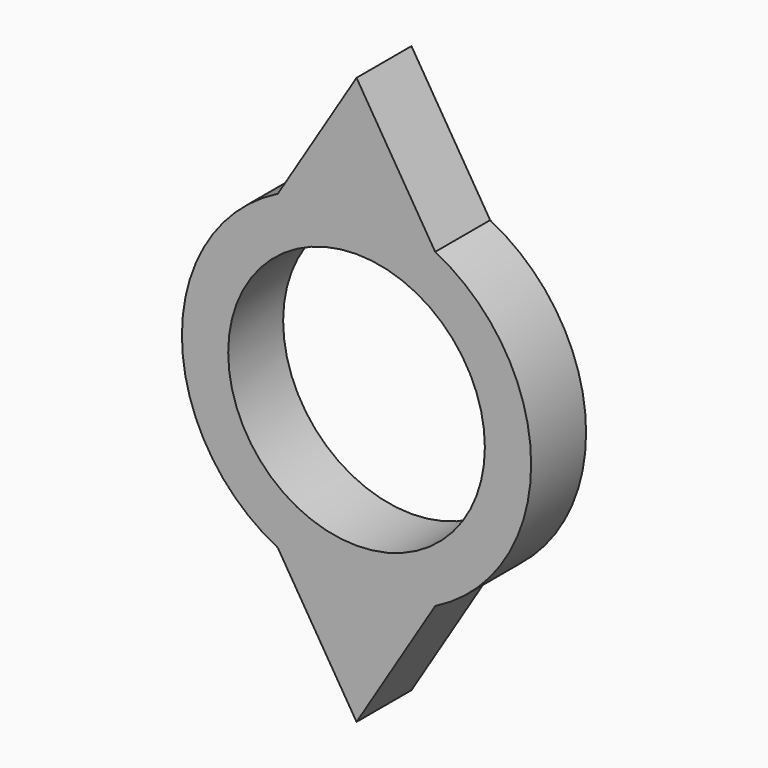
from build123d import *

# Parameters (mm, degrees)
F0_R     = 15
F0_R_2   = 11.025
F3_DEPTH = 25
F2_R     = 11.025
F4_DEPTH = 40.1
F6_DEPTH = 15
F7_DEPTH = 7
F8_DEPTH = 2.9


# Not quite as in the source:
# - ends of sketch curves that miss each other by under 0.0002 mm in the source are joined


with BuildPart() as f3:
    # F0 (on Front) → F3 (new body)
    with BuildSketch(Plane.XZ):
        Circle(F0_R)
        Circle(F0_R_2, mode=Mode.SUBTRACT)
    extrude(amount=F3_DEPTH)


with BuildPart() as f3b:
    # F1 (on Front) → F3, piece 2 (new body)
    with BuildSketch(Plane.XZ):
        Polygon((0, 24.356296724), (-6.821225702, 13.2896405025), (-6.821225702, 0), (0, 0), (6.821225702, 0), (6.821225702, 13.2896405025), align=None)
        Polygon((0, 0), (-6.821225702, 0), (-6.821225702, -10.4577671736), (-6.82123, -10.4854255915), (-6.821225702, -13.2896405025), (0, -24.356296724), (6.821225702, -13.2896405025), (6.821225702, 0), align=None)
    extrude(amount=F3_DEPTH)

    # F2 (on face) → F4 (cut)
    with BuildSketch(Plane.XZ):
        Circle(F2_R)
    extrude(amount=F4_DEPTH, mode=Mode.SUBTRACT)

    # F5: union F3
    add(f3.part)

    # F6 (cut): a face of the model
    f6_faces = [f3b.faces().sort_by_distance(p)[0] for p in [
        (-11.5970941147, -25, 0),
    ]]
    extrude(f6_faces, amount=-F6_DEPTH, mode=Mode.SUBTRACT)

    # F7 (cut): a face of the model
    f7_faces = [f3b.faces().sort_by_distance(p)[0] for p in [
        (-11.5970941147, 0, 0),
    ]]
    extrude(f7_faces, amount=-F7_DEPTH, mode=Mode.SUBTRACT)

    # F8 (add): a face of the model
    f8_faces = [f3b.faces().sort_by_distance(p)[0] for p in [
        (-11.5970941147, -10, 0),
    ]]
    extrude(f8_faces, amount=F8_DEPTH)


solid = f3b.part
